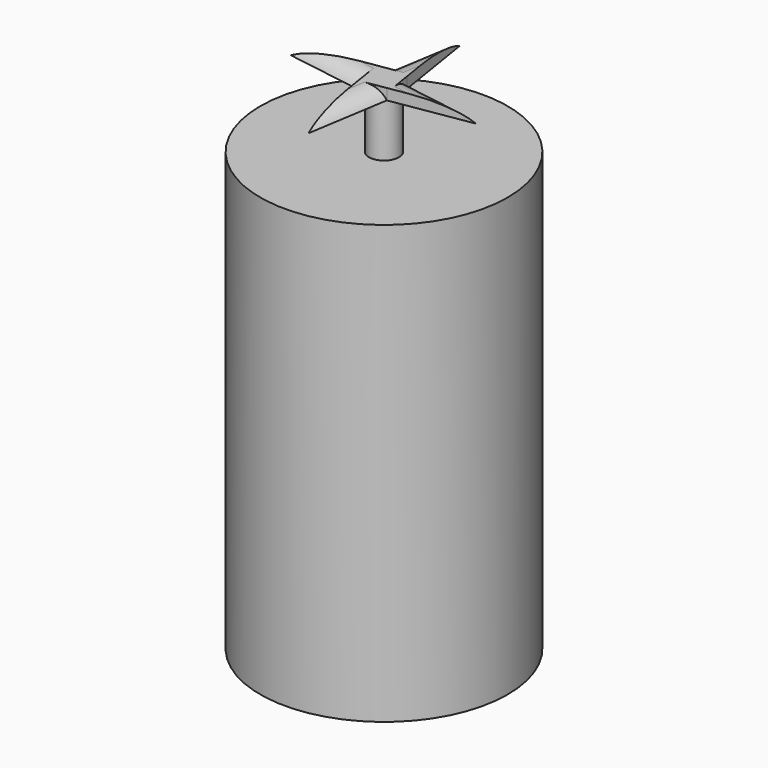
from build123d import *

# Parameters (mm, degrees)
F0_R         = 28.7287455722
F1_DEPTH     = 101.6
F2_R         = 3.4611907446
F3_DEPTH     = 12.7
F5_DEPTH     = 2.54
F6_T4_DEPTH  = 41.1832125644
F6_T9_DEPTH  = 40.5629822974
F6_T14_DEPTH = 41.203398669
F6_T19_DEPTH = 40.8847394673


# Not quite as in the source:
# - a fillet or chamfer that OpenCascade refuses, or shapes differently, is made with other operations: its cross-section is extruded or revolved along the edge and cut away or added


with BuildPart() as f1:
    # F0 (on Top) → F1 (new body)
    with BuildSketch(Plane.XY):
        Circle(F0_R)
    extrude(amount=F1_DEPTH)

    # F2 (on face) → F3 (join)
    with BuildSketch(Plane.XY.offset(101.6)):
        Circle(F2_R)
    extrude(amount=F3_DEPTH)

    # F4 (on face) → F5 (join)
    with BuildSketch(Plane.XY.offset(114.3)):
        Polygon((-2.9900876214, -2.9829602297), (-3.4611907446, 0), (-2.9961511649, 2.9445667062), (-21.6407428614, 0), align=None)
        Polygon((-2.9961511649, 2.9445667062), (-3.4611907446, 0), (-2.9900876214, -2.9829602297), (0, -3.4611907446), (3.0300985076, -2.9704015808), (3.5051804641, 0), (3.0362172662, 2.9321446653), (0, 3.4177530923), align=None)
        Polygon((0, 21.9157841057), (-2.9961511649, 2.9445667062), (0, 3.4177530923), (3.0362172662, 2.9321446653), align=None)
        Polygon((0, -3.4611907446), (-2.9900876214, -2.9829602297), (0, -21.9157841057), (3.0300985076, -2.9704015808), align=None)
        Polygon((21.3691533617, 0), (3.0362172662, 2.9321446653), (3.5051804641, 0), (3.0300985076, -2.9704015808), align=None)
    extrude(amount=F5_DEPTH)

    # F6: fillet of radius 5.08 on 4 edges, made by hand


with BuildPart() as f6_tool2:
    # F6_s3 → F6_t4 (new body)
    with BuildSketch(Plane(origin=(-5.1547653088, -32.2296454573, 0), x_dir=(0, 0, 1), z_dir=(0.1579314127, 0.9874500842, 0))):
        with BuildLine():
            ThreePointArc((116.84, -0.9382183066), (116.1594090512, 1.6017816934), (114.3, 3.4611907446))
            Line((114.3, 3.4611907446), (116.84, 3.4611907446))
            Line((116.84, 3.4611907446), (116.84, -0.9382183066))
        make_face()
    extrude(amount=F6_T4_DEPTH)

    split(bisect_by=Plane(origin=(0.5462821974, -3.3727086764, 0), x_dir=(0, 0, 1), z_dir=(0.1598876303, -0.9871352216, 0)), keep=Keep.TOP)


with BuildPart() as f1_1:
    add(f1.part)

    # F6_t1: cut F6_tool2
    add(f6_tool2.part, mode=Mode.SUBTRACT)


with BuildPart() as f6_tool7:
    # F6_s8 → F6_t9 (new body)
    with BuildSketch(Plane(origin=(31.6966489584, -5.0695185795, 0), x_dir=(0, 0, 1), z_dir=(-0.9874500842, 0.1579314127, 0))):
        with BuildLine():
            ThreePointArc((116.84, -1.0245484723), (116.1594090512, 1.5154515277), (114.3, 3.374860579))
            Line((114.3, 3.374860579), (116.84, 3.374860579))
            Line((116.84, 3.374860579), (116.84, -1.0245484723))
        make_face()
    extrude(amount=F6_T9_DEPTH)

    split(bisect_by=Plane(origin=(3.4177530923, 0.546630744, 0), x_dir=(0, 0, 1), z_dir=(0.9874500842, 0.1579314127, 0)), keep=Keep.TOP)


with BuildPart() as f1_2:
    add(f1_1.part)

    # F6_t6: cut F6_tool7
    add(f6_tool7.part, mode=Mode.SUBTRACT)


with BuildPart() as f6_tool12:
    # F6_s13 → F6_t14 (new body)
    with BuildSketch(Plane(origin=(5.0927080964, 32.2463277493, 0), x_dir=(0, 0, 1), z_dir=(-0.155997919, -0.9877573838, 0))):
        with BuildLine():
            ThreePointArc((116.84, -0.9805923365), (116.1594090512, 1.5594076635), (114.3, 3.4188167147))
            Line((114.3, 3.4188167147), (116.84, 3.4188167147))
            Line((116.84, 3.4188167147), (116.84, -0.9805923365))
        make_face()
    extrude(amount=F6_T14_DEPTH)

    split(bisect_by=Plane(origin=(-0.5266350679, 3.3345808721, 0), x_dir=(0, 0, 1), z_dir=(-0.155997919, 0.9877573838, 0)), keep=Keep.TOP)


with BuildPart() as f1_3:
    add(f1_2.part)

    # F6_t11: cut F6_tool12
    add(f6_tool12.part, mode=Mode.SUBTRACT)


with BuildPart() as f6_tool17:
    # F6_s18 → F6_t19 (new body)
    with BuildSketch(Plane(origin=(-31.9614643829, 5.1118727954, 0), x_dir=(0, 0, 1), z_dir=(0.9874500842, -0.1579314127, 0))):
        with BuildLine():
            ThreePointArc((114.3, 3.4177530923), (116.1594090512, 1.5583440411), (116.84, -0.9816559589))
            Line((116.84, -0.9816559589), (116.84, 3.4177530923))
            Line((116.84, 3.4177530923), (114.3, 3.4177530923))
        make_face()
    extrude(amount=F6_T19_DEPTH)

    split(bisect_by=Plane(origin=(-3.3769614538, -0.5333282931, 0), x_dir=(0, 0, 1), z_dir=(-0.9877573838, -0.155997919, 0)), keep=Keep.TOP)


with BuildPart() as f1_4:
    add(f1_3.part)

    # F6_t16: cut F6_tool17
    add(f6_tool17.part, mode=Mode.SUBTRACT)


solid = f1_4.part
